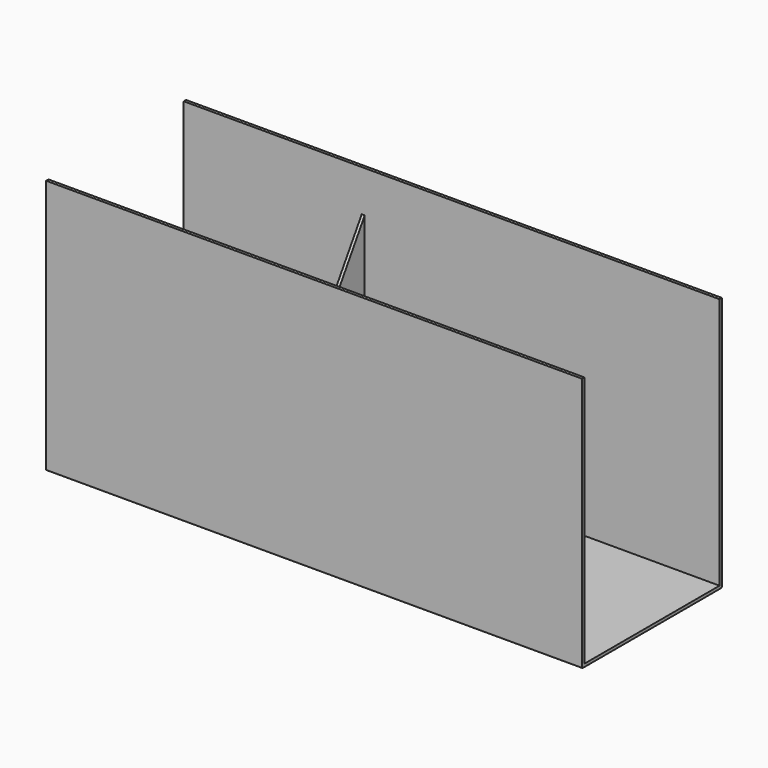
from build123d import *

# Parameters (mm, degrees)
F1_DEPTH = 903
F4_DEPTH = 5
F5_R     = 2


# Not quite as in the source:
# - a feature names something its author has since deleted; it is built from what else it names


with BuildPart() as f1:
    # F0 (on Right) → F1 (new body)
    with BuildSketch(Plane.YZ):
        Polygon((-295, 0), (0, 0), (0, 430), (-5, 430), (-5, 5), (-290, 5), (-290, 430), (-295, 430), align=None)
    extrude(amount=F1_DEPTH)

    # F3 (on offset) → F4 (join)
    with BuildSketch(Plane.YZ.offset(300)):
        Polygon((-230, 0), (-5, 0), (-5, 360), align=None)
    extrude(amount=F4_DEPTH)

    # F5
    f5_edges = [f1.edges().sort_by_distance(p)[0] for p in [
        (451.5, 0, 0),
        (451.5, -295, 0),
    ]]
    fillet(f5_edges, radius=F5_R)


solid = f1.part
